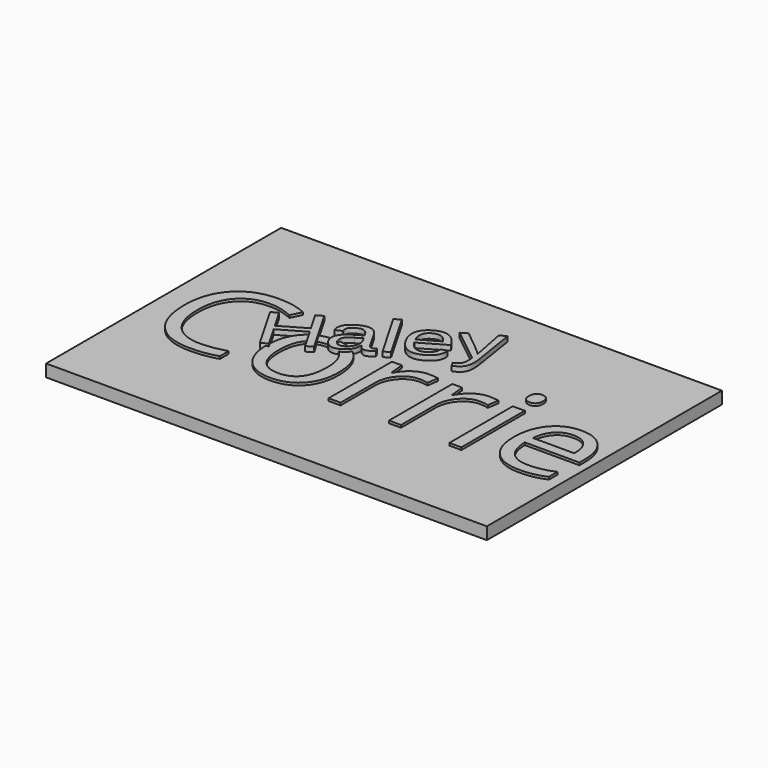
from build123d import *

# Parameters (mm, degrees)
F0_TEXT_SIZE = 153.4862538184
F1_DEPTH     = 2.54
F2_W         = 457.2
F2_H         = 304.8
F3_DEPTH     = 12.7
F5_TEXT_SIZE = 79.5400611621
F6_DEPTH     = 5.08
F8_ANGLE     = 330


# Not quite as in the source:
# - Text() gives the source's letters only with a copy of the font that has no kerning and outlines rounded to 1/6400 em; it was checked with that copy


with BuildPart() as f1:
    # F0 (on Top) → F1 (new body)
    with BuildSketch(Plane.XY):
        with Locations((-84.5386459795, -51.1058324534)):
            Text('Corrie', F0_TEXT_SIZE, font='Open Sans', text_align=(TextAlign.LEFT, TextAlign.BOTTOM))
    extrude(amount=F1_DEPTH)


with BuildPart() as f3:
    # F2 (on Top) → F3 (new body)
    with BuildSketch(Plane.XY):
        with Locations((228.6, 9.7513739711)):
            Rectangle(F2_W, F2_H)
    extrude(amount=F3_DEPTH)


with BuildPart() as f1_1:
    # F4: moved
    add(f1.part.moved(Location((101.6, 0, 12.7))))


with BuildPart() as f6:
    # F5 (on Top) → F6 (new body)
    with BuildSketch(Plane.XY):
        with Locations((8.2970588151, -14.3265296944)):
            Text('Haley', F5_TEXT_SIZE, font='Arimo', text_align=(TextAlign.LEFT, TextAlign.BOTTOM))
    extrude(amount=F6_DEPTH)


with BuildPart() as f6_1:
    # F7: moved
    add(f6.part.moved(Location((152.4, -76.2, 12.7))))


with BuildPart() as f6_2:
    # F8: moved
    add(f6_1.part.rotate(Axis((0, -142.6486260289, 6.35), (0, 0, -1)), F8_ANGLE))


solid = Compound([f3.part, f1_1.part, f6_2.part])
